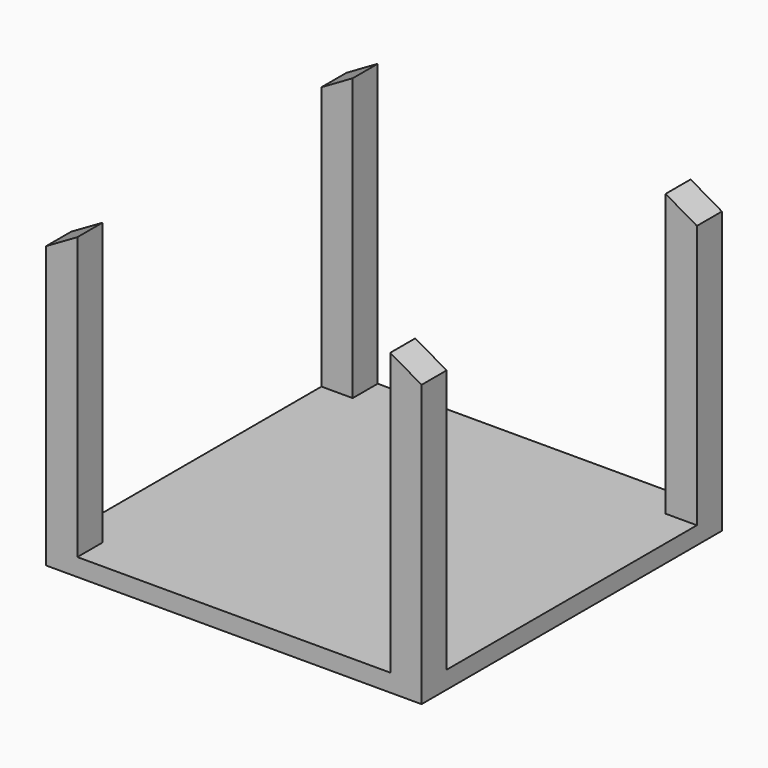
from build123d import *

# Parameters (mm, degrees)
F0_W          = 1219.2
F0_H          = 1219.2
F1_DEPTH      = 19.05
F2_W          = 1219.2
F2_H          = 1219.2
F2_W_2        = 1041.4
F2_H_2        = 476.25
F3_DEPTH      = 38.1
F4_W          = 101.6
F4_H          = 101.6
F5_DEPTH      = 914.4
F7_DEPTH      = 2867
F7_DEPTH_BACK = 1219.201


# Not quite as in the source:
# - an extrude ends at something that could not be found from the text; its depth is read off the source's solid


with BuildPart() as f1:
    # F0 (on Top) → F1 (new body)
    with BuildSketch(Plane.XY):
        with Locations((609.6, 609.6)):
            Rectangle(F0_W, F0_H)
    extrude(amount=F1_DEPTH)

    # F2 (on face) → F3 (join)
    with BuildSketch(Plane(origin=(0, 0, 0), x_dir=(1, 0, 0), z_dir=(0, 0, -1))):
        with Locations((609.6, -609.6)):
            Rectangle(F2_W, F2_H)
        with Locations((609.6, -892.175)):
            Rectangle(F2_W_2, F2_H_2, mode=Mode.SUBTRACT)
        with Locations((609.6, -327.025)):
            Rectangle(F2_W_2, F2_H_2, mode=Mode.SUBTRACT)
    extrude(amount=F3_DEPTH)

    # F4 (on face) → F5 (join)
    with BuildSketch(Plane.XY.offset(19.05)):
        with Locations((50.8, 1168.4)):
            Rectangle(F4_W, F4_H)
        with Locations((50.8, 50.8)):
            Rectangle(F4_W, F4_H)
        with Locations((1168.4, 50.8)):
            Rectangle(F4_W, F4_H)
        with Locations((1168.4, 1168.4)):
            Rectangle(F4_W, F4_H)
    extrude(amount=F5_DEPTH)

    # F6 (on face) → F7 (cut, two sides)
    with BuildSketch(Plane.XZ) as f7_sk:
        Polygon((0, 874.7912126503), (101.6, 933.45), (0, 933.45), align=None)
        Polygon((1219.2, 933.45), (1117.6, 933.45), (1219.2, 874.7912126503), align=None)
    extrude(amount=F7_DEPTH, mode=Mode.SUBTRACT)
    extrude(f7_sk.sketch, amount=-F7_DEPTH_BACK, mode=Mode.SUBTRACT)


solid = f1.part
